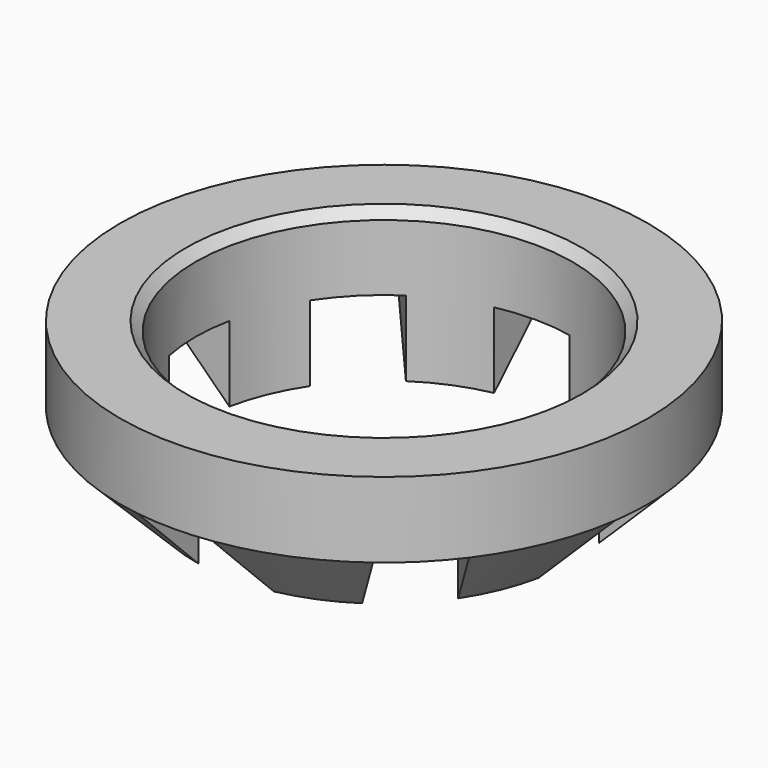
from build123d import *

# Parameters (mm, degrees)
F0_R            = 14
F0_R_2          = 10
F1_DEPTH        = 4
F2_R            = 14
F2_R_2          = 10
F3_DEPTH        = 4
F4_SIZE         = 0.5
F5_SIZE         = 3.99999
F6_W            = 4
F6_H            = 40
F7_DEPTH        = 4.001
F7_COPIES_COUNT = 4
F7_COPIES_ANGLE = 135


# Not quite as in the source:
# - a fillet or chamfer is up to 0.001 mm smaller than in the source, because OpenCascade refuses the exact size
# - a pattern or mirror of a feature is missing from the dataset's text; its kind, count and spacing are read off the source's solid


with BuildPart() as f1:
    # F0 (on Top) → F1 (new body)
    with BuildSketch(Plane.XY):
        Circle(F0_R)
        Circle(F0_R_2, mode=Mode.SUBTRACT)
    extrude(amount=F1_DEPTH)

    # F2 (on face) → F3 (join)
    with BuildSketch(Plane(origin=(0, 0, 0), x_dir=(1, 0, 0), z_dir=(0, 0, -1))):
        Circle(F2_R)
        Circle(F2_R_2, mode=Mode.SUBTRACT)
    extrude(amount=F3_DEPTH)

    # F4
    f4_edges = [f1.edges().sort_by_distance(p)[0] for p in [
        (-10, 0, 4),
    ]]
    chamfer(f4_edges, length=F4_SIZE)

    # F5 (size 4 in the source; OpenCascade refuses exactly that, so slightly less here)
    f5_edges = [f1.edges().sort_by_distance(p)[0] for p in [
        (-14, 0, -4),
    ]]
    chamfer(f5_edges, length=F5_SIZE)

    # F6 (on Top) → F7 (cut, through all)
    with BuildSketch(Plane.XY):
        Rectangle(F6_W, F6_H)
    f7 = extrude(amount=-F7_DEPTH, mode=Mode.SUBTRACT)

    # F7_copies: F7 ×4 about axis
    f7_copies_axis = Axis((0, 0, 0), (0, 0, 1))
    for i in range(1, F7_COPIES_COUNT):
        add(f7.rotate(f7_copies_axis, i * F7_COPIES_ANGLE / (F7_COPIES_COUNT - 1)), mode=Mode.SUBTRACT)


solid = f1.part
